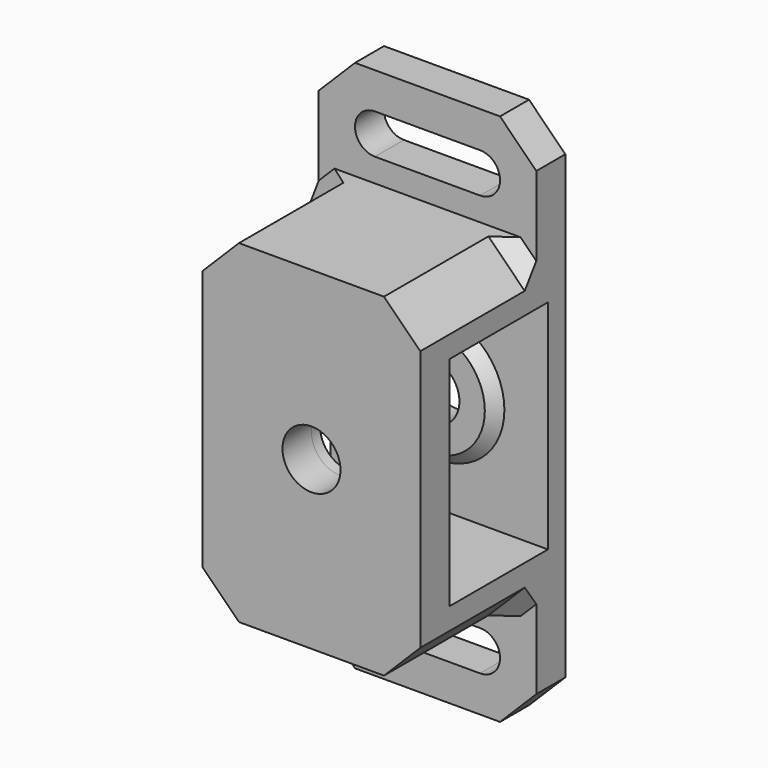
from build123d import *

# Parameters (mm, degrees)
F0_R     = 11
F0_R_2   = 4
F1_DEPTH = 3
F0_W     = 30
F0_H     = 8
F2_DEPTH = 20
F3_DEPTH = 5
F4_W     = 30
F4_H     = 46
F4_R     = 4
F5_DEPTH = 5
F6_R     = 7
F6_R_2   = 4
F7_DEPTH = 1.5
F8_R     = 7
F8_R_2   = 4
F9_DEPTH = 1.5
F10_SIZE = 5
F12_SIZE = 2


# Not quite as in the source:
# - a fillet or chamfer that OpenCascade refuses, or shapes differently, is made with other operations: its cross-section is extruded or revolved along the edge and cut away or added


with BuildPart() as f1:
    # F0 (on Front) → F1 (new body)
    with BuildSketch(Plane.XZ):
        Polygon((15, 15), (-15, 15), (-15, 0), (-15, -15), (15, -15), (15, 0), align=None)
        Circle(F0_R, mode=Mode.SUBTRACT)
        Circle(F0_R)
        Circle(F0_R_2, mode=Mode.SUBTRACT)
    extrude(amount=F1_DEPTH)

    # F0 (on Front) → F2 (join)
    with BuildSketch(Plane.XZ):
        with Locations((0, 19)):
            Rectangle(F0_W, F0_H)
        with Locations((0, -19)):
            Rectangle(F0_W, F0_H)
    extrude(amount=F2_DEPTH)

    # F0 (on Front) → F3 (join)
    with BuildSketch(Plane.XZ):
        Polygon((15, -23), (-15, -23), (-15, -36.75), (0, -36.75), (15, -36.75), align=None)
        with BuildLine():
            ThreePointArc((-7.25, -31.75), (-10, -29), (-7.25, -26.25))
            Line((-7.25, -26.25), (7.25, -26.25))
            ThreePointArc((7.25, -26.25), (10, -29), (7.25, -31.75))
            Line((7.25, -31.75), (-7.25, -31.75))
        make_face(mode=Mode.SUBTRACT)
        Polygon((-15, 36.75), (-15, 23), (15, 23), (15, 36.75), (0, 36.75), align=None)
        with BuildLine():
            ThreePointArc((-7.25, 26.25), (-10, 29), (-7.25, 31.75))
            Line((-7.25, 31.75), (7.25, 31.75))
            ThreePointArc((7.25, 31.75), (10, 29), (7.25, 26.25))
            Line((7.25, 26.25), (-7.25, 26.25))
        make_face(mode=Mode.SUBTRACT)
    extrude(amount=F3_DEPTH)

    # F4 (on face) → F5 (join)
    with BuildSketch(Plane.XZ.offset(20)):
        Rectangle(F4_W, F4_H)
        Circle(F4_R, mode=Mode.SUBTRACT)
    extrude(amount=F5_DEPTH)

    # F6 (on face) → F7 (join)
    with BuildSketch(Plane.XZ.offset(3)):
        Circle(F6_R)
        Circle(F6_R_2, mode=Mode.SUBTRACT)
    extrude(amount=F7_DEPTH)

    # F8 (on face) → F9 (join)
    with BuildSketch(Plane(origin=(0, -20, 0), x_dir=(-1, 0, 0), z_dir=(0, 1, 0))):
        Circle(F8_R)
        Circle(F8_R_2, mode=Mode.SUBTRACT)
    extrude(amount=F9_DEPTH)

    # F10
    f10_edges = [f1.edges().sort_by_distance(p)[0] for p in [
        (15, -2.5, 36.75),
        (-15, -2.5, 36.75),
        (15, -2.5, -36.75),
        (-15, -2.5, -36.75),
        (-15, -15, 23),
        (15, -15, 23),
        (15, -15, -23),
        (-15, -15, -23),
    ]]
    chamfer(f10_edges, length=F10_SIZE)

    # F11: chamfer of 2 on 2 edges, made by hand


with BuildPart() as f11_tool2:
    # F11_s3 → F11_t4 (revolve)
    with BuildSketch(Plane.XY):
        Polygon((9, -3), (7, -5), (7, -3), align=None)
    revolve(axis=Axis((0, -3, 0), (0, -1, 0)))

    split(bisect_by=Plane.XZ.offset(4.5), keep=Keep.BOTTOM)


with BuildPart() as f1_1:
    add(f1.part)

    # F11_t1: union F11_tool2
    add(f11_tool2.part)


with BuildPart() as f11_tool7:
    # F11_s8 → F11_t9 (revolve)
    with BuildSketch(Plane.XY):
        Polygon((-9, -20), (-7, -18), (-7, -20), align=None)
    revolve(axis=Axis((0, -20, 0), (0, 1, 0)))

    split(bisect_by=Plane.XZ.offset(18.5), keep=Keep.TOP)


with BuildPart() as f1_2:
    add(f1_1.part)

    # F11_t6: union F11_tool7
    add(f11_tool7.part)

    # F12
    f12_edges = [f1_2.edges().sort_by_distance(p)[0] for p in [
        (12.5, -5, 20.5),
        (-12.5, -5, 20.5),
        (-12.5, -5, -20.5),
        (12.5, -5, -20.5),
    ]]
    chamfer(f12_edges, length=F12_SIZE)


solid = f1_2.part
